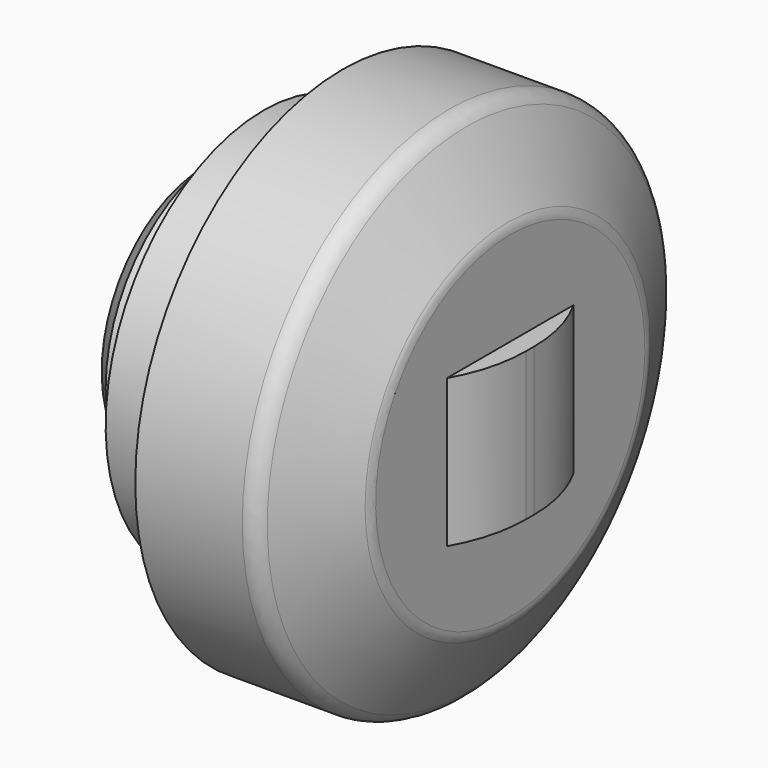
from build123d import *

# Parameters (mm, degrees)
F3_SIZE     = 2
F4_SIZE2    = 8.6602540378
F4_SIZE     = 5
F5_R        = 2
F6_W        = 16
F6_H        = 15
F7_DEPTH    = 2
F8_T1_DEPTH = 52.4165738677


# Not quite as in the source:
# - a fillet or chamfer that OpenCascade refuses, or shapes differently, is made with other operations: its cross-section is extruded or revolved along the edge and cut away or added


with BuildPart() as f2:
    # F0 (on Front) → F2 (revolve)
    with BuildSketch(Plane.XZ):
        Polygon((0, 15), (0, 0), (31, 0), (31, 26.25), (14, 26.25), (14, 20), (6, 20), (6, 15), align=None)
    revolve(axis=Axis((43.7085926533, 0, 0), (1, 0, 0)))

    # F3
    f3_edges = [f2.edges().sort_by_distance(p)[0] for p in [
        (0, 0, -15),
    ]]
    chamfer(f3_edges, length=F3_SIZE)

    # F4
    f4_edges = [f2.edges().sort_by_distance(p)[0] for p in [
        (31, 0, -26.25),
    ]]
    chamfer(f4_edges, length=F4_SIZE, length2=F4_SIZE2)

    # F5
    f5_edges = [f2.edges().sort_by_distance(p)[0] for p in [
        (26, 0, -26.25),
        (31, 0, -17.589746),
    ]]
    fillet(f5_edges, radius=F5_R)

    # F6 (on face) → F7 (join)
    with BuildSketch(Plane.YZ.offset(31)):
        Rectangle(F6_W, F6_H)
    extrude(amount=F7_DEPTH)

    # F8: fillet of radius 15 on 2 edges, made by hand

    # F8_s2 → F8_t1 (cut)
    with BuildSketch(Plane.XY.offset(-26.2082869339)):
        with BuildLine():
            ThreePointArc((31, -8), (32.4913767462, -4.3896685727), (33, -0.5166852265))
            Line((33, -0.5166852265), (33, -8))
            Line((33, -8), (31, -8))
        make_face()
        with BuildLine():
            ThreePointArc((31, 8), (32.4913767462, 4.3896685727), (33, 0.5166852265))
            Line((33, 0.5166852265), (33, 8))
            Line((33, 8), (31, 8))
        make_face()
    extrude(amount=F8_T1_DEPTH, mode=Mode.SUBTRACT)


solid = f2.part
